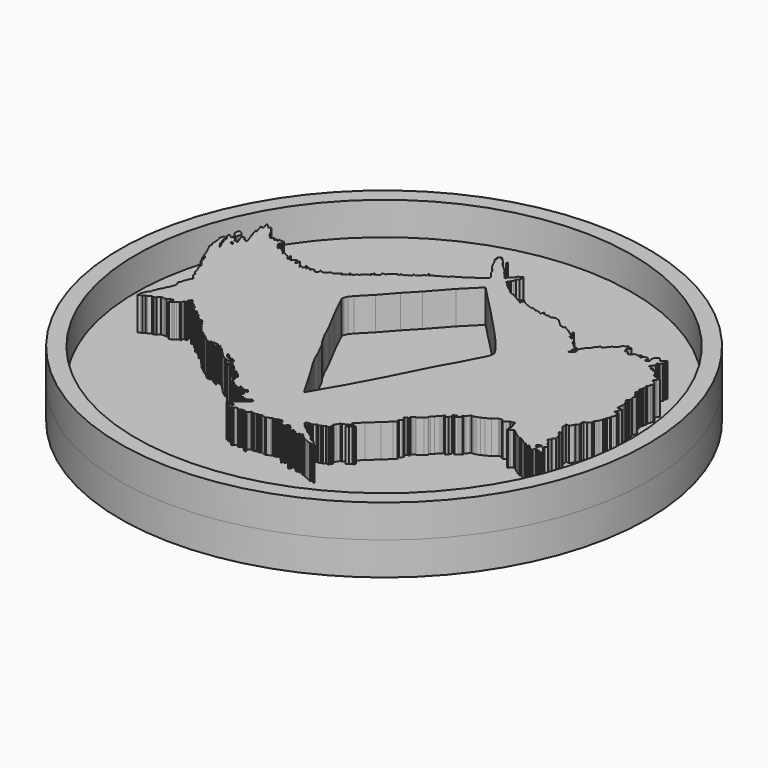
from build123d import *

# Parameters (mm, degrees)
F1_DEPTH = 2.5
F2_R     = 20
F2_R_2   = 18.8
F3_DEPTH = 2.5
F4_DEPTH = 2.5


with BuildPart() as f1:
    # F0 (on Top) → F1 (new body)
    with BuildSketch(Plane.XY):
        Polygon((2.8794382233, -10.7436152175), (2.8547642287, -10.5685461313), (2.8042409103, -10.7001410797), (2.7466679458, -10.7788639143), (2.7513678651, -10.8258621767), (2.7830917388, -10.8658103272), (2.835964784, -10.8705107123), (2.8770884965, -10.8364364132), (2.9052873142, -10.7906134799), align=None)
    extrude(amount=F1_DEPTH)


with BuildPart() as f1b:
    # F0 (on Top) → F1, piece 2 (new body)
    with BuildSketch(Plane.XY):
        Polygon((4.7097317874, -9.2714289203), (4.6033868566, -9.4176540151), (4.7296718694, -9.3312487006), (4.8094303347, -9.311308153), (4.9357153475, -9.1783767566), (5.0420602784, -9.1717308387), (5.1085259765, -9.0255057439), (4.9822414294, -9.0853255242), (4.9024824984, -9.1451443732), (4.7296718694, -9.1451443732), align=None)
    extrude(amount=F1_DEPTH)


with BuildPart() as f1c:
    # F0 (on Top) → F1, piece 3 (new body)
    with BuildSketch(Plane.XY):
        Polygon((2.7880056296, 9.804864414), (2.7621455956, 9.796067141), (2.7610280085, 9.7378306091), (2.7869136538, 9.7201569006), (2.831000369, 9.7271725535), (2.8474458959, 9.7436271608), (2.8180237859, 9.7701279446), (2.8097650502, 9.7977844998), align=None)
    extrude(amount=F1_DEPTH)


with BuildPart() as f1d:
    # F0 (on Top) → F1, piece 4 (new body)
    with BuildSketch(Plane.XY):
        Polygon((0.836121093, 10.7127986848), (0.8675596328, 10.6785539538), (0.9017927223, 10.6652751565), (0.9325326537, 10.6764575467), (0.9388203616, 10.7114007697), (0.9003954474, 10.7596227899), (0.842408801, 10.7596227899), align=None)
    extrude(amount=F1_DEPTH)


with BuildPart() as f1e:
    # F0 (on Top) → F1, piece 5 (new body)
    with BuildSketch(Plane.XY):
        Polygon((-1.0246526217, 12.8345778212), (-0.9706045967, 12.7852298319), (-0.9142065537, 12.7993291244), (-0.9165564552, 12.8392782062), (-0.9447555058, 12.8815760836), (-0.9447555058, 12.9191754386), (-0.9612049325, 12.9520744085), (-1.0035034502, 12.9497237504), (-1.0246526217, 12.9191754386), align=None)
    extrude(amount=F1_DEPTH)


with BuildPart() as f1f:
    # F0 (on Top) → F1, piece 6 (new body)
    with BuildSketch(Plane.XY):
        Polygon((-14.5434308797, 0.128211148), (-14.492415823, 0), (-14.3880443648, -0.1093972533), (-14.3209751695, -0.1149863165), (-14.3042076379, -0.1513153402), (-14.2622897401, -0.2239733585), (-14.2790572718, -0.3161931236), (-14.3628930673, -0.3720839159), (-14.3740717322, -0.475481851), (-14.4355511293, -0.6152088172), (-14.5193869248, -0.7884702063), (-14.5333595574, -0.9673206951), (-14.5764509216, -1.0409364477), (-14.6416602656, -1.1239300948), (-14.657468535, -1.1970434571), (-14.6495644003, -1.2780609541), (-14.5744746551, -1.3669827022), (-14.5329786465, -1.4598564012), (-14.5468106493, -1.5072813258), (-14.5626189187, -1.6139873769), (-14.615971595, -1.7187173944), (-14.6653726697, -1.8866806058), (-14.7167500108, -2.015122911), (-14.7878872231, -2.0585958846), (-14.8234562948, -2.2463193163), (-14.9084255099, -2.428114647), (-15.038844198, -2.5921256747), (-15.0783648714, -2.7245201636), (-15.0924259797, -2.8712532949), (-15.1289822534, -2.8579602949), (-15.1622146368, -2.8313740622), (-15.2020948008, -2.8513136785), (-15.1588916779, -3.017477924), (-15.1921240613, -3.1437624712), (-15.3383491561, -3.2833404839), (-15.3782283887, -3.3365131821), (-15.4181076214, -3.4860610031), (-15.5277764425, -3.635608824), (-15.4912201688, -3.7220141385), (-15.5011899769, -3.8383293431), (-15.5477160588, -3.9014716167), (-15.5443921685, -3.9479974657), (-15.4912201688, -3.9745839313), (-15.3649346903, -3.8782085758), (-15.2353271842, -3.8383293431), (-15.1223354042, -3.7087211385), (-15.0525458157, -3.6954279058), (-14.9960499257, -3.6854580976), (-14.7401569411, -3.5458800849), (-14.6770151332, -3.5624965094), (-14.6072255448, -3.5757897422), (-14.5174972713, -3.5359102767), (-14.4610013813, -3.4960308112), (-14.4277680665, -3.429565113), (-14.3181001768, -3.3331897575), (-14.2649272457, -3.2866639085), (-14.1153791919, -3.2833404839), (-14.0156811103, -3.2999569084), (-13.8694560155, -3.2866639085), (-13.6999692768, -3.1271460466), (-13.6401494965, -3.1304694712), (-13.6069171131, -3.1736721285), (-13.5570680723, -3.1637023203), (-13.5038951412, -3.1105296221), (-13.4440762922, -3.1204996631), (-13.4174898267, -3.1603788957), (-13.4141659364, -3.2235214021), (-13.4341064841, -3.2401378267), (-13.4407524019, -3.3298665658), (-13.5603910312, -3.4495047294), (-13.5304816067, -3.4760911949), (-13.3842565119, -3.3797158394), (-13.3344074711, -3.3464829903), (-13.2180927321, -3.3066035248), (-13.1350103766, -3.2334912103), (-13.0552519113, -3.1470858958), (-12.995432131, -3.087266814), (-12.9522299394, -3.0939131975), (-12.9322903231, -3.1271460466), (-12.9057038575, -3.1736721285), (-12.8525309265, -3.1603788957), (-12.8724705428, -3.0939131975), (-12.9057038575, -3.0407407321), (-12.8957340494, -2.9709516093), (-12.8458840773, -2.8679298703), (-12.7727724612, -2.8513134457), (-12.7428630367, -2.8978395276), (-12.7495089546, -2.9343955684), (-12.6558227235, -2.9278331026), (-12.593314983, -2.8679298703), (-12.6066077501, -2.7482914738), (-12.6597806811, -2.7549380902), (-12.7096297219, -2.7715545148), (-12.7395391464, -2.7449682821), (-12.7362161875, -2.6785025839), (-12.6996599138, -2.6186835021), (-12.6631036401, -2.5455711875), (-12.6099316403, -2.4957219139), (-12.5833451748, -2.449195832), (-12.5334952027, -2.4558424484), (-12.4969398603, -2.4890752975), (-12.4836461619, -2.5356013793), (-12.5235253945, -2.5389245711), (-12.5368190929, -2.5655108038), (-12.593314983, -2.5887738448), (-12.6199014485, -2.6220066939), (-12.593314983, -2.6352999266), (-12.5268492848, -2.631976502), (-12.5102326274, -2.6087134611), (-12.4305552999, -2.6058834381), (-12.3673314229, -2.6718562003), (-12.2144604102, -2.8313738294), (-12.1413478628, -2.8446670622), (-12.1081154794, -2.8778999113), (-12.1114384383, -2.9144559521), (-12.1546406299, -2.9709518421), (-12.1878739446, -3.017477924), (-12.1347010136, -3.064003773), (-12.1347010136, -3.1337928958), (-12.1147613972, -3.1537325121), (-12.0715592057, -3.1271462794), (-12.0449727401, -3.0507107731), (-11.9884768501, -2.9842450749), (-11.935303919, -2.9775984585), (-11.8721621111, -3.0540339649), (-11.8688382208, -3.1603791285), (-11.81898918, -3.246784443), (-11.7359068245, -3.3298665658), (-11.6528244689, -3.3996556886), (-11.5830358118, -3.4162721131), (-11.5464795381, -3.4362117294), (-11.5198930725, -3.4694445785), (-11.4866606891, -3.462798195), (-11.4999534562, -3.3930090722), (-11.4667210728, -3.3863624558), (-11.3636991009, -3.5060008522), (-11.2573541701, -3.5757897422), (-11.2772937864, -3.6555486731), (-11.3238198683, -3.7253377959), (-11.2939104438, -3.7851568777), (-11.2507073209, -3.7751868367), (-11.1975343898, -3.7186911795), (-11.1643020064, -3.7419542205), (-11.1410384998, -3.7652170286), (-11.0878665, -3.7652170286), (-11.0945133492, -3.7153677549), (-11.0612800345, -3.6954281386), (-11.0247237608, -3.7286609877), (-11.0180769116, -3.7652170286), (-11.0546331853, -3.7785102613), (-11.0579570755, -3.828359535), (-10.9914913774, -3.8748856168), (-11.0014611855, -3.9247348905), (-10.9017621726, -3.9513208903), (-10.8552360907, -3.9745839313), (-10.7854474336, -4.0476964787), (-10.762183927, -4.1208085604), (-10.6757786125, -4.2238305323), (-10.5926971883, -4.3202056549), (-10.5594638735, -4.3002660386), (-10.6026669964, -4.203890916), (-10.6093129143, -4.1374252178), (-10.5694336817, -4.0942225605), (-10.5262314901, -4.1008689441), (-10.473058559, -4.1540414095), (-10.3933000937, -4.180627875), (-10.3633897379, -4.2304769158), (-10.3301573545, -4.3334988877), (-10.260367766, -4.4398442842), (-10.1340832189, -4.5661288314), (-10.1565420628, -4.5993616804), (-10.1565420628, -4.6658483334), (-10.1012121886, -4.699440673), (-10.01821924, -4.7290814109), (-9.9846264347, -4.8002186231), (-9.8127108067, -5.0412951969), (-9.6091795713, -5.2369232289), (-9.5222331583, -5.2566835657), (-9.2080431059, -5.5333287455), (-9.1151697561, -5.5590169504), (-8.9116375893, -5.7329083793), (-8.6389444768, -5.9720091522), (-8.5974484682, -5.9720091522), (-8.5816401988, -5.9384163469), (-8.5381669924, -5.9403921477), (-8.484814316, -5.9897932224), (-8.4294844419, -5.9917694889), (-8.3823278546, -5.8678621426), (-8.3212293684, -5.872562062), (-8.3212293684, -5.9618586674), (-8.2648312673, -5.9665585868), (-8.1943338737, -5.8631622232), (-8.1285368651, -5.8584623039), (-8.0721378326, -5.914860405), (-8.0674383789, -5.9665585868), (-8.1097371876, -5.990057718), (-8.0909375101, -6.0605555773), (-8.001640439, -6.1451522633), (-7.8324470669, -6.2297494151), (-7.7337501571, -6.2908474356), (-7.7055511065, -6.2532485463), (-7.80894747, -6.0934540816), (-7.9828416929, -5.9383595362), (-7.9828416929, -5.9007611126), (-7.8653451055, -5.9007611126), (-7.8183468431, -5.9618586674), (-7.7337501571, -5.9994575568), (-7.6726521365, -6.0746548697), (-7.6323859394, -6.0681444593), (-7.6519171707, -5.9752599336), (-7.6116649434, -5.9836371802), (-7.5837196782, -6.0115824454), (-7.5390068814, -6.1177751049), (-7.3936907575, -6.1568985693), (-6.9968663156, -6.564901676), (-6.7118234001, -6.855533924), (-6.4491364174, -7.0455623791), (-6.3429442234, -7.1405768394), (-6.3094096258, -7.0790969767), (-6.0858465731, -7.1797003038), (-5.7999179699, -7.1964673698), (-5.5309436284, -7.3802778497), (-5.5260532536, -7.4194013141), (-5.5309436284, -7.4410592206), (-5.6119854562, -7.4389632791), (-5.653903354, -7.4655115604), (-5.709095858, -7.4704019353), (-5.7356436737, -7.4508399703), (-5.7649863884, -7.4061276391), (-5.7999179699, -7.4054286815), (-5.8292606845, -7.4277850799), (-5.8306581341, -7.5451559387), (-5.8250688016, -7.6003479771), (-5.7831509039, -7.6338825747), (-5.7272603735, -7.6303891838), (-5.6755612604, -7.605238352), (-5.6455200538, -7.5940601528), (-5.6301504374, -7.6101287268), (-5.571465008, -7.6799923554), (-5.5057932623, -7.7309925109), (-5.4603819735, -7.7344859019), (-5.4338336922, -7.7156224288), (-5.4345326498, -7.6632248238), (-5.4834363982, -7.621306926), (-5.54771116, -7.5500458479), (-5.5183684453, -7.5214020908), (-5.4750530981, -7.5144157745), (-5.3758467548, -7.512319833), (-5.3444080986, -7.5430595316), (-5.3139394149, -7.5977724046), (-5.249904003, -7.6606324874), (-5.1688319072, -7.7240802348), (-5.1406333223, -7.7693159692), (-5.0836475566, -7.8803496435), (-5.0025759265, -7.9884454608), (-4.9614524469, -8.0043077469), (-4.9326657318, -8.0184070393), (-4.9203289673, -8.0372067168), (-4.9044666812, -8.0389687791), (-4.8909545876, -8.0213444307), (-4.8850798048, -7.972584106), (-4.8551186919, -7.9396851361), (-4.8175198026, -7.9379221424), (-4.792845808, -7.9561341554), (-4.778158851, -8.0107701942), (-4.7975103371, -8.0780889839), (-4.8377527855, -8.1048198044), (-4.8565519974, -8.1059942022), (-4.8853382468, -8.0963009968), (-4.907369148, -8.0713331699), (-4.936743062, -8.0836704001), (-4.9438299611, -8.1195728853), (-4.9047064967, -8.139135316), (-4.8390347511, -8.1796552986), (-4.770568572, -8.2243680954), (-4.7230613418, -8.2634920254), (-4.6378280967, -8.3221774548), (-4.5623756014, -8.3976294845), (-4.5022927225, -8.4674935788), (-4.486923106, -8.5150003433), (-4.4533885084, -8.5122054443), (-4.4491966255, -8.4730824456), (-4.4575803913, -8.4185888991), (-4.503690172, -8.35012272), (-4.5595807023, -8.2844505087), (-4.6434169635, -8.202011697), (-4.7202669084, -8.1377374008), (-4.7188694589, -8.0762580037), (-4.6559926122, -8.0748600885), (-4.6294443309, -8.0874357373), (-4.5861289836, -8.139135316), (-4.503690172, -8.2257660106), (-4.4422103092, -8.277464658), (-4.3667578138, -8.3529166877), (-4.3360176496, -8.422780782), (-4.3304287829, -8.5122054443), (-4.3541821651, -8.5303699598), (-4.3835248798, -8.5331648588), (-4.4277254492, -8.552370593), (-4.4158692472, -8.5997954011), (-4.3714088388, -8.6156036705), (-4.3299118988, -8.6521608755), (-4.3200314976, -8.7035372853), (-4.3177357875, -8.746878244), (-4.3529844843, -8.751578629), (-4.3882331811, -8.7163290009), (-4.6349745244, -8.511886932), (-4.7877193429, -8.4413895383), (-4.9827625044, -8.2815950736), (-5.0274110399, -8.2839448005), (-5.0274110399, -8.3191934973), (-4.8464671709, -8.4766382352), (-4.6725734137, -8.5823843256), (-4.3703098781, -8.8347969577), (-4.3021366, -8.8476408273), (-4.2695323937, -8.8812336326), (-4.2626159266, -8.925694041), (-4.2952205986, -8.9622503147), (-4.2892927304, -9.0264715254), (-4.2398916557, -9.0610524639), (-4.1578859091, -9.0808132663), (-4.0986048989, -9.1163814068), (-3.9019891992, -9.2942258343), (-3.8259117864, -9.3149738386), (-3.7972591817, -9.3623986468), (-3.7942952476, -9.5007214695), (-3.7607026752, -9.5343142748), (-3.7172297016, -9.5293736085), (-3.6866010632, -9.4938054681), (-3.6895652302, -9.4483559951), (-3.7201938685, -9.4177275896), (-3.6698048934, -9.3940151855), (-3.6115117837, -9.4157522544), (-3.5275302362, -9.470093064), (-3.4484886564, -9.511590004), (-3.3674712759, -9.5679070801), (-3.2983098645, -9.5738349482), (-3.3081900328, -9.5382668078), (-3.3546269406, -9.4750327989), (-3.4020519815, -9.4078481197), (-3.4554048907, -9.3367109075), (-3.447500756, -9.2784175649), (-3.4010638483, -9.2803938314), (-3.3733993769, -9.3080578372), (-3.3338784706, -9.3495547771), (-3.3220222685, -9.3910517171), (-3.3368426375, -9.4384765252), (-3.3210343681, -9.470093064), (-3.2825015951, -9.470093064), (-3.2676812261, -9.4335367903), (-3.2874417957, -9.3801831827), (-3.2745974604, -9.3218907714), (-3.2370528206, -9.3544945121), (-3.214328317, -9.4167403877), (-3.1688795425, -9.4592245296), (-3.1619633082, -9.4888648018), (-3.1787597109, -9.5135653391), (-3.1836999115, -9.5600029454), (-3.1491192058, -9.5955710858), (-3.1184905674, -9.5679070801), (-3.1145385001, -9.5155416057), (-3.078969894, -9.478985332), (-3.0295688193, -9.4681167975), (-3.0107966159, -9.4434162602), (-2.9604076408, -9.4513203949), (-2.9554674402, -9.4809606671), (-2.922863001, -9.4918292016), (-2.8922343627, -9.4671286643), (-2.884330228, -9.4197038561), (-2.8457974549, -9.3762306497), (-2.7904682793, -9.3821594492), (-2.7446213644, -9.4327088445), (-2.7105624322, -9.4983885065), (-2.662953455, -9.553863667), (-2.6595285162, -9.6027906984), (-2.6643229648, -9.6385413781), (-2.7136956342, -9.6389073879), (-2.7333348989, -9.6118757501), (-2.7759657241, -9.5736039802), (-2.812409075, -9.5619810745), (-2.8387901839, -9.5730004832), (-2.8639938682, -9.5964064822), (-2.8681331314, -9.6304118633), (-2.8318210971, -9.6573270857), (-2.7942510787, -9.6872197464), (-2.7833986096, -9.7675379366), (-2.7471387293, -9.800334461), (-2.691736212, -9.8442640156), (-2.6922437828, -9.9030807614), (-2.7167205699, -9.9165057763), (-2.7269828133, -9.9915200844), (-2.7566659264, -10.013859719), (-2.7942019515, -10.0545044988), (-2.7952319942, -10.0997332484), (-2.7659838088, -10.1283127442), (-2.7263986412, -10.1476246491), (-2.6645348407, -10.185437277), (-2.6564844884, -10.2190319449), (-2.6371406857, -10.2809742093), (-2.5919666514, -10.3209223598), (-2.5399958249, -10.3163029999), (-2.4642604403, -10.2701280266), (-2.42394628, -10.2839870378), (-2.4239073973, -10.3422887623), (-2.4388970342, -10.3924917057), (-2.4225749075, -10.4381563142), (-2.3956054356, -10.436527431), (-2.3880430963, -10.3723956272), (-2.3656536359, -10.3390868753), (-2.330571413, -10.3345969692), (-2.3125640582, -10.3718852624), (-2.2290314082, -10.3759253398), (-2.2109330166, -10.3400908411), (-2.1629389375, -10.3387329727), (-2.1405748557, -10.3711355478), (-2.0698797889, -10.363153182), (-1.9555764738, -10.2994069457), (-1.896721893, -10.2260541171), (-1.8758515362, -10.1818563417), (-1.8310520099, -10.1755158976), (-1.7952256603, -10.2100688964), (-1.780948136, -10.2423671633), (-1.7529044999, -10.2412458509), (-1.7392452573, -10.2201765403), (-1.7106310697, -10.2156046778), (-1.6968038399, -10.2304108441), (-1.6927962424, -10.2660348639), (-1.6669204924, -10.2663682774), (-1.6629811144, -10.3098973632), (-1.6974124592, -10.3015489876), (-1.7234585248, -10.3209763765), (-1.6977177002, -10.3371180594), (-1.702507725, -10.3923929855), (-1.7546651652, -10.4391528293), (-1.87175069, -10.5127431452), (-1.932838466, -10.5949612334), (-2.0933183841, -10.6996148825), (-2.2541387007, -10.843789205), (-2.4408134632, -10.9487883747), (-2.5386204943, -11.0405934975), (-2.6165654417, -11.1426245421), (-2.6530593168, -11.168744415), (-2.6650137734, -11.1885322258), (-2.6334433351, -11.2072201446), (-2.5782184675, -11.2170716748), (-2.5484983344, -11.2407198176), (-2.5269410107, -11.2642636523), (-2.5344947353, -11.2990653142), (-2.5692218915, -11.3310245797), (-2.616596641, -11.3570038229), (-2.6545650326, -11.3440509886), (-2.7051893994, -11.3267805427), (-2.7573485859, -11.2762534991), (-2.8253407218, -11.2753771245), (-2.8591775335, -11.3090099767), (-2.8569214046, -11.3630490378), (-2.815447282, -11.3901728764), (-2.7519909199, -11.3918213174), (-2.6829980779, -11.3819083199), (-2.6343241334, -11.41577214), (-2.6230842341, -11.4790676162), (-2.5888672099, -11.5069290623), (-2.5434782729, -11.5008661523), (-2.4657761678, -11.4270830527), (-2.4158682209, -11.3421399146), (-2.3665726185, -11.3361282274), (-2.3199392017, -11.3209402189), (-2.2916600574, -11.3196428865), (-2.2644661367, -11.3391047344), (-2.2610439919, -11.365737766), (-2.274771221, -11.3713778555), (-2.3088706657, -11.4141469821), (-2.3202942684, -11.4713348448), (-2.309355652, -11.5794958547), (-2.2741658613, -11.6239888594), (-2.2062866483, -11.6846896708), (-2.1950600203, -11.7587875575), (-2.1678581834, -11.7774177343), (-2.1230611019, -11.7638697848), (-2.0963505376, -11.7326378822), (-2.0829422865, -11.656364426), (-2.0379344933, -11.6178914905), (-1.9482675707, -11.5824844688), (-1.7986700404, -11.5769337863), (-1.7790239071, -11.626210995), (-1.7375795869, -11.685741134), (-1.7186414916, -11.7109129205), (-1.6866568476, -11.7030153051), (-1.6800557496, -11.6773415357), (-1.6165057896, -11.6025451571), (-1.5781818656, -11.5997148678), (-1.5469130594, -11.5685435012), (-1.4283066848, -11.5617616102), (-1.4226280618, -11.5369064733), (-1.3916689204, -11.5422913805), (-1.3910334092, -11.5747051314), (-1.3666915474, -11.6082550958), (-1.3376430143, -11.623586528), (-1.3317067642, -11.5688210353), (-1.3259297702, -11.5323355421), (-1.2940651504, -11.5385623649), (-1.2915447587, -11.5643525496), (-1.2644589879, -11.5962773561), (-1.2034100946, -11.6020496935), (-1.1999645503, -11.6261914372), (-1.2420060812, -11.6372834891), (-1.2823358411, -11.6616915911), (-1.2764462736, -11.7199318483), (-1.2519740267, -11.7376977578), (-1.2157390593, -11.7664150894), (-1.1751411948, -11.8184564635), (-1.1380241485, -11.8505088612), (-1.0972052114, -11.8759628385), (-1.0562147945, -11.8814762682), (-1.0114887264, -11.876235716), (-0.9903045138, -11.8515808135), (-0.9909097571, -11.8150124326), (-1.0191196343, -11.8080014363), (-1.1096363887, -11.7278974503), (-1.0833578417, -11.6401575506), (-1.058412483, -11.6022555158), (-1.0243271245, -11.5611478686), (-0.9774729842, -11.5202050656), (-0.9389062179, -11.4882960916), (-0.9221833316, -11.4519502968), (-0.9200038039, -11.4096011966), (-0.8934841026, -11.400802061), (-0.8561364957, -11.4054372534), (-0.833510072, -11.4256711677), (-0.8410406299, -11.4538259804), (-0.8495628717, -11.4911077544), (-0.8169547655, -11.517287232), (-0.7504168316, -11.5206371993), (-0.6844786694, -11.4874178544), (-0.4738125717, -11.485144496), (-0.4214989603, -11.4451032132), (-0.3647063277, -11.4150904119), (-0.3384963202, -11.4428484812), (-0.3223508538, -11.4746317267), (-0.2886975708, -11.4850364625), (-0.257655367, -11.4804506302), (-0.2455709036, -11.4531852305), (-0.2161066514, -11.419496499), (-0.1647239551, -11.3819353282), (-0.0762701166, -11.3822445273), (-0.0345674307, -11.4110326394), (-0.0128800957, -11.4345774055), (0.0872699093, -11.453316547), (0.1590794564, -11.4808315411), (0.2412182512, -11.4727495238), (0.3274827613, -11.40821632), (0.4711195361, -11.353562586), (0.5765866372, -11.2826293334), (0.6623227964, -11.2804099917), (0.6876258412, -11.3073261455), (0.7323202444, -11.3062402233), (0.7553371834, -11.2799461931), (0.7784797344, -11.239528656), (0.81944064, -11.2483650446), (0.8393296157, -11.2685644999), (0.8794008754, -11.2748965621), (0.9114962304, -11.2537061796), (0.8834143518, -11.2317400053), (0.8610110381, -11.1849196255), (0.8765882812, -11.1759798601), (0.9139775066, -11.1756306142), (0.9777678642, -11.1806066707), (0.9931360837, -11.1965918913), (1.0340771405, -11.2079214305), (1.0724719614, -11.1967828125), (1.1148686754, -11.1433193088), (1.1677107541, -11.148984544), (1.2001374271, -11.1967660487), (1.3040129561, -11.2064126879), (1.3326881453, -11.2666077912), (1.3347847853, -11.3422498107), (1.2959734304, -11.3642485812), (1.2959734304, -11.4032393321), (1.3130656444, -11.4308791235), (1.3769947691, -11.4572355524), (1.4075816143, -11.4674111828), (1.4332249993, -11.5180499852), (1.4667029027, -11.5492260084), (1.4879414812, -11.5767493844), (1.4929594472, -11.6180386394), (1.5073154354, -11.6433771327), (1.5316131758, -11.6716390476), (1.546653104, -11.7067694664), (1.5720090596, -11.7008071393), (1.5770804603, -11.6449743509), (1.5568216331, -11.5923089907), (1.5441527357, -11.5488255396), (1.5612980351, -11.5162059665), (1.5874719247, -11.5039655939), (1.6103740782, -11.5161389112), (1.6045932425, -11.5649756044), (1.6342197778, -11.598196812), (1.6856824514, -11.5883797407), (1.7479301896, -11.5724112839), (1.7750544939, -11.5385232493), (1.7848344287, -11.4701744169), (1.8258518539, -11.4252846688), (1.8499820726, -11.3829728216), (1.8967994256, -11.3779865205), (1.9149947912, -11.402675882), (1.9532544538, -11.412252672), (1.9755812827, -11.4013608545), (1.9903734792, -11.3749988377), (2.0194663666, -11.3802654669), (2.0369400736, -11.4000542089), (2.0458565559, -11.4337084815), (2.0725447685, -11.4515200257), (2.0714821294, -11.4864427596), (2.0429727156, -11.5028452128), (2.0433743484, -11.546170339), (2.0568773616, -11.5812812001), (2.0873788744, -11.6019360721), (2.1430081688, -11.6431796923), (2.1669236012, -11.6260191426), (2.1153187845, -11.5624694154), (2.1193204448, -11.5422578529), (2.1599882748, -11.5392878652), (2.1766899154, -11.559067294), (2.2093774751, -11.5930270404), (2.2128811106, -11.7230350152), (2.2585373372, -11.7648486048), (2.2982556839, -11.7828277871), (2.3539855611, -11.8121933192), (2.3988650646, -11.8553936481), (2.3983621504, -11.9147794321), (2.3751542903, -11.9389351457), (2.3460180964, -11.9385598227), (2.3083202541, -11.9534470141), (2.3034969345, -11.9799356908), (2.3170770146, -12.0059633628), (2.3769652471, -11.9969528168), (2.4027100299, -11.9448797777), (2.4257835466, -11.9367921725), (2.4737427011, -11.8871014565), (2.469797153, -11.8094924837), (2.445789054, -11.7949787527), (2.4499809369, -11.7488689721), (2.482118085, -11.7069510743), (2.5659543462, -11.7090465501), (2.5959955528, -11.749567464), (2.6414068416, -11.7803076282), (2.7147633955, -11.7831015959), (2.7594761923, -11.8201291189), (2.776941983, -11.8536641821), (2.8020928148, -11.9053637609), (2.8502985369, -11.9563639164), (2.9089839663, -11.9975833222), (2.9809433036, -11.9968848303), (3.0039981939, -11.9731305167), (3.0158751179, -11.9207333773), (3.0508066993, -11.8858013302), (3.0759575311, -11.8396915495), (3.1213688198, -11.828513816), (3.1597937923, -11.8348011747), (3.16887605, -11.8592530489), (3.136738902, -11.8823079392), (3.100409871, -11.9214318693), (3.140930552, -11.9731305167), (3.1968213152, -11.9598563761), (3.2191777136, -11.8927871808), (3.2897398341, -11.8438834324), (3.2799588516, -11.8138417602), (3.2436300535, -11.7810061201), (3.3079043496, -11.7726223543), (3.3735760953, -11.8501707911), (3.3945350442, -11.9333080947), (3.5022012889, -11.9918836281), (3.4528530668, -12.0388818905), (3.4575529862, -12.0788309723), (3.5022012889, -12.1023301035), (3.5562494304, -12.0388818905), (3.600897966, -12.0435822755), (3.600897966, -12.0905805379), (3.683145158, -12.1634276584), (3.7324933801, -12.175177224), (4.0779314004, -12.330272235), (4.1719279252, -12.3467212543), (4.2330259457, -12.4031193554), (4.3364223093, -12.4524673447), (4.4327690266, -12.389020063), (4.7006593086, -12.5182652846), (4.7147590667, -12.4971158803), (4.5526148751, -12.3373214155), (4.4025308453, -12.1875908226), (4.286557436, -12.0702199638), (4.2460365221, -12.0296990499), (4.2125023901, -11.9975619018), (4.2013241909, -12.0324939489), (4.1901459917, -12.0841925964), (4.0769670159, -12.028302066), (4.0085008368, -11.9752055034), (3.927459009, -11.8690133095), (3.8883355446, -11.8159167469), (3.8841438945, -11.6985458881), (3.9218701422, -11.669203639), (3.9260620251, -11.6230938584), (3.8939246442, -11.6077233106), (3.8464176469, -11.6356695071), (3.8296503481, -11.6831762716), (3.7360333372, -11.6747925058), (3.6466079764, -11.6147100925), (3.5753473639, -11.5420520306), (3.3112633973, -11.3953389227), (3.1617556233, -11.2500227988), (3.0863031279, -11.1745707691), (2.9898914509, -11.1298579723), (2.8906853404, -11.0613917932), (2.8753154911, -11.0250627622), (2.9088498559, -10.9901307151), (2.89627444, -10.9076919034), (2.8417808935, -10.9160756692), (2.815232845, -10.9649803489), (2.7691230644, -10.9663773328), (2.7230130509, -10.9314452857), (2.6573413052, -10.8420206234), (2.6238069404, -10.7428142801), (2.5525460951, -10.7232527807), (2.4575316347, -10.6128687039), (2.4673126172, -10.53322386), (2.5427651126, -10.4661546648), (2.6349849068, -10.4382093996), (2.6852865703, -10.394894518), (2.7272047009, -10.3976884857), (2.7313965838, -10.4396063834), (2.7383829001, -10.5583751574), (2.7579446323, -10.5835255235), (2.787287347, -10.5583751574), (2.8040546458, -10.4857170954), (2.8669317253, -10.4200448841), (2.9004660901, -10.4200448841), (2.9144389555, -10.4493880644), (2.9675350524, -10.4451961815), (3.1212347094, -10.2803185582), (3.1980846543, -10.2621540427), (3.2176463865, -10.3096608073), (3.2875097822, -10.3040719405), (3.3881133422, -10.2230301127), (3.4551820718, -10.2188382298), (3.4761412535, -10.2453865111), (3.5725529306, -10.2286189795), (3.6759506911, -10.1028652862), (3.7625813857, -10.0860977545), (3.833842231, -10.1419882849), (3.8827466778, -10.1280156523), (3.8869385608, -10.0805088878), (3.9330483414, -10.0218234584), (3.9274594747, -9.9491653964), (4.00291197, -9.9449735135), (4.0238709189, -9.890479967), (3.9484184235, -9.8164249212), (3.8967193104, -9.718616493), (3.8995139766, -9.6515472978), (4.0126927197, -9.5537388697), (4.1440362111, -9.3231890351), (4.250228405, -9.3176001683), (4.4081201777, -9.2058181763), (4.4360654429, -9.2700924724), (4.5254910365, -9.182064794), (4.6386695467, -9.1024199501), (4.7434647568, -9.0968310833), (4.7797937877, -9.0493233874), (4.7197113745, -9.0185841545), (4.6749985777, -8.9235696942), (4.7079001818, -8.7904037561), (5.206303671, -8.3300461993), (5.9009861243, -7.6702110477), (6.4279139042, -7.1835066192), (6.610956043, -7.014437113), (6.6025727428, -6.9424775429), (6.5529695712, -6.9026555866), (6.5543670207, -6.7943669856), (6.7080669105, -6.6672158428), (6.7499848083, -6.6106263548), (6.755573675, -6.5142144449), (6.5941894427, -6.4240903594), (6.6004772671, -6.3716927543), (6.7674508318, -6.2508285046), (6.8687526509, -6.2389518134), (6.9253421389, -6.1795678921), (6.9393147714, -6.1586089432), (6.9148628972, -6.1404444277), (6.847793702, -6.1229784042), (6.8554785103, -6.0817589983), (6.9064791314, -6.0461289249), (6.9546848536, -5.9727719054), (7.0534395054, -5.9045953676), (7.1260975674, -5.8682663366), (7.1579422802, -5.9026554227), (7.5341002084, -5.6167580187), (7.693388965, -5.4714418948), (7.7269230969, -5.3904005326), (7.6654432341, -5.3680441342), (7.6654432341, -5.33730397), (7.7353068627, -5.2730296738), (7.916951552, -5.1333028823), (8.1385448575, -4.8903045245), (8.2278419286, -4.801007919), (8.2912901416, -4.7023114748), (8.3594378084, -4.6647125855), (8.4205353633, -4.6811620705), (8.4369843826, -4.725810606), (8.4134852514, -4.7916080803), (8.4698833525, -4.8057078384), (8.5192322731, -4.7775087878), (8.6273280904, -4.6882117167), (8.6555276066, -4.6059647575), (8.6954757571, -4.5519163832), (8.7166251615, -4.4626197778), (8.6884256452, -4.3968218379), (8.6672771722, -4.3310243636), (8.8035715744, -4.2511271313), (8.911668323, -4.213528242), (8.9563168585, -4.2323279195), (8.9234178886, -4.2981253937), (8.8693695143, -4.4062216766), (8.8623203337, -4.4649695046), (8.9234178886, -4.4626197778), (9.0855611488, -4.3427739292), (9.1678090394, -4.2581767775), (9.2947045341, -4.1735796258), (9.3088038266, -4.1359812021), (9.2571051791, -4.138330929), (9.2077571899, -4.1477307677), (9.1748582199, -4.138330929), (9.1490093619, -4.1030822322), (9.1560594738, -4.0537337773), (9.2030577362, -3.9996858686), (9.3581518158, -3.9174389094), (9.4826975837, -3.7576442119), (9.5743443817, -3.689496778), (9.7435377538, -3.6847968586), (9.8915826529, -3.6377985962), (10.135974735, -3.5532014444), (10.3850653395, -3.4357055556), (10.7399029657, -3.2477120403), (11.0571421683, -2.9821712524), (11.12058945, -2.9586721212), (11.2451352179, -2.9657220002), (11.3132828847, -2.9539722018), (11.367331259, -2.9892211314), (11.3861300051, -3.0409193132), (11.4049296826, -3.0714680906), (11.4613277838, -3.0879175756), (11.5200756118, -3.0738180503), (11.6258217022, -2.9915710911), (11.7715168744, -2.8693752829), (11.8373148143, -2.8341265861), (11.9900591671, -2.836476313), (12.1028553694, -2.8247267473), (12.1545530856, -2.7871280909), (12.1898027137, -2.7988776565), (12.1921524405, -2.8388262726), (12.1639529243, -2.9210734647), (12.1663026512, -2.9986207373), (12.2415004298, -3.0244698282), (12.2908484191, -3.1701647677), (12.3448967934, -3.3229093533), (12.3495962471, -3.4780038986), (12.3002482578, -3.499153303), (12.264999561, -3.5673007369), (12.3448967934, -3.656597808), (12.3448967934, -3.7834933028), (12.3848449439, -3.8328415249), (12.4388933182, -3.8187419996), (12.4647421762, -3.7435446866), (12.5234900042, -3.6683473736), (12.6456860453, -3.5837502219), (12.7091342583, -3.557901131), (12.7678820863, -3.574350616), (12.8853777424, -3.6824468989), (13.0992205814, -3.8492910098), (13.2754640654, -3.9691366255), (13.5151557624, -4.1148317978), (13.5927032679, -4.1430308484), (13.6232515797, -4.1312812828), (13.6937499046, -4.1265813634), (13.9006730169, -4.2631248944), (14.0753323212, -4.401454702), (14.2010860145, -4.4587426819), (14.2639633268, -4.4769071974), (14.3264252692, -4.4465810061), (14.346987009, -4.4689052738), (14.3483411521, -4.4816131704), (14.4155258313, -4.5606545173), (14.4649269059, -4.5863431878), (14.5163042471, -4.6159834601), (14.5854651928, -4.6258638613), (14.6407941356, -4.5487983152), (14.6803148091, -4.5784390531), (14.7672602907, -4.6396963298), (14.8522304371, -4.7503542155), (14.9826491252, -4.8155635595), (15.0715708733, -4.8985569738), (15.1268998161, -4.8689167015), (15.1348039508, -4.7701145522), (15.1427080855, -4.6495762654), (15.1664204895, -4.5883189887), (15.2355814353, -4.5883189887), (15.2869587764, -4.6159834601), (15.3225269169, -4.6535283327), (15.3561197221, -4.6772407368), (15.4193527997, -4.6811928041), (15.5161786824, -4.7266418114), (15.5774364248, -4.764186684), (15.6189324334, -4.8096352257), (15.6545024365, -4.8116114922), (15.6703107059, -4.7878990881), (15.6861189753, -4.764186684), (15.6999509782, -4.8116114922), (15.7710872591, -4.7681387514), (15.7453995198, -4.6495762654), (15.7118067145, -4.5744869858), (15.545819886, -4.3749068864), (15.4648022726, -4.3057459407), (15.4252815992, -4.256344866), (15.4151087627, -4.1462080553), (15.4715068638, -4.1368086822), (15.6360007823, -4.0099127218), (15.5937029049, -3.915916197), (15.377510339, -3.7561217323), (15.3305120766, -3.6527253687), (15.2459153906, -3.5117303487), (15.1801174507, -3.4130339045), (15.0908203796, -3.3848348539), (15.0250224397, -3.3331366722), (15.0156235322, -3.2720386516), (15.0720207021, -3.2062411774), (15.1715520769, -3.1211215537), (15.1250259951, -3.0745954718), (15.0917936116, -3.02806939), (15.1715520769, -2.981543541), (15.3310699388, -2.8619051445), (15.1914916933, -2.4431713391), (15.0851467624, -2.2903000936), (14.9854486808, -2.2238343954), (14.9189829826, -2.1573686972), (14.9721549824, -2.0842563827), (15.051914379, -2.0709631499), (15.1250259951, -2.0443769172), (15.0386206806, -1.8981524045), (14.6597661078, -1.4195992844), (14.666412957, -1.3066076208), (14.6797057241, -1.2202021899), (14.6398264915, -1.1537363753), (14.6597661078, -1.0872706771), (14.7195858881, -1.0739775607), (14.8791028187, -1.0806241771), (15.0585602969, -0.8413475589), (15.0917936116, -0.7150627207), (15.1724535972, -0.644225569), (15.2674680576, -0.5548003246), (15.2339339256, -0.4541969392), (15.2115775272, -0.3759497777), (15.289824456, -0.2865245333), (15.2339339256, -0.2474010398), (15.2618791908, -0.174743036), (15.4574969783, -0.1244412706), (15.5413327739, -0.0182488347), (15.6195806339, 0.0544091672), (15.6810600311, 0.0935327407), (15.7201830298, 0.2276706073), (15.6810600311, 0.2444378624), (15.6698822975, 0.272383244), (15.7034154981, 0.2891504846), (15.7648958266, 0.3618084884), (15.8599112183, 0.5462480476), (15.9772820771, 0.7586330175), (15.9325692803, 0.7865783991), (15.9213896841, 0.8312910213), (16.0164050758, 0.9263053653), (16.0164050758, 1.1051559122), (16.1337759346, 1.2169374386), (16.1058306694, 1.3622534461), (16.1952544004, 1.4908022713), (16.2679124624, 1.6025837976), (16.3126252592, 1.66965276), (16.2902697921, 1.7423107056), (16.2455569953, 1.7255435232), (16.1728989333, 1.7478998052), (16.1784887314, 1.8149687676), (16.2064339966, 1.8764486304), (16.1561314017, 1.9379284931), (16.1617211998, 2.0105864387), (16.0275828093, 1.9770520739), (15.8766768873, 1.9658738747), (15.8375538886, 2.0049973391), (15.9493349493, 2.1503134631), (15.9925278276, 2.3548081517), (16.0489268601, 2.4582045153), (15.9502308816, 2.4535048287), (15.8985313028, 2.5334020611), (15.8280339092, 2.4958034046), (15.7152377069, 2.4629044347), (15.6823396683, 2.5381017476), (15.6964398921, 2.7871930506), (15.7340373844, 2.9610870406), (15.7011393458, 3.10678198), (15.6588405371, 3.2289775554), (15.6400408596, 3.2994751818), (15.687039122, 3.332373919), (15.6917385757, 3.4216709901), (15.7528370619, 3.4216709901), (15.7951358706, 3.4686692525), (15.7622359693, 3.5485664848), (15.6964398921, 3.572065616), (15.6212411821, 3.5250673536), (15.5460443348, 3.4733691718), (15.4849467799, 3.4874686971), (15.4708465561, 3.5532664042), (15.536644496, 3.6284637172), (15.6212411821, 3.7318600807), (15.6353414059, 3.8352564443), (15.6053351238, 3.96407675), (15.5630363151, 4.0157749318), (15.5865354463, 4.0674731135), (15.5959352851, 4.1802693158), (15.6382340938, 4.2648664676), (15.661733225, 4.354163073), (15.6288351864, 4.3823621236), (15.5724361539, 4.3682628311), (15.5395371839, 4.3353638612), (15.5160380527, 4.3729622848), (15.506638214, 4.4481600635), (15.4549404979, 4.4481600635), (15.4032418504, 4.4951583259), (15.4173420742, 4.5844549313), (15.3844431043, 4.6549527906), (15.3045458719, 4.6361531131), (15.271646902, 4.6831518412), (15.2951460332, 4.7348500229), (15.3186451644, 4.7959475778), (15.3421442956, 4.8805447295), (15.3186451644, 4.9698418006), (15.3233446181, 5.0591384061), (15.2481477708, 5.0638383254), (15.2481477708, 5.1014372148), (15.271646902, 5.1296362653), (15.2763463557, 5.2001336589), (15.2904465795, 5.3082299419), (15.3280450031, 5.3552282043), (15.3515441343, 5.3928266279), (15.3186451644, 5.4210256785), (15.3182623908, 5.4731206037), (15.3322350234, 5.509449169), (15.3769478202, 5.601669196), (15.3713589534, 5.6827110238), (15.309878625, 5.6407926604), (15.273549594, 5.637998227), (15.2987008914, 5.7386015542), (15.3713589534, 5.8475886472), (15.4076879844, 5.9593701735), (15.4412221164, 6.0655628331), (15.4887298122, 6.1577823944), (15.4831400141, 6.2416186556), (15.424455516, 6.3226600178), (15.3266461566, 6.4316471107), (15.2707556263, 6.5015107393), (15.2148650959, 6.4987163059), (15.1785360649, 6.4735654742), (15.1394121349, 6.4903325401), (15.1505898684, 6.5853470005), (15.2600212023, 6.7459307611), (15.300530009, 6.8091638386), (15.3855001554, 6.8812891841), (15.3489429504, 6.9089536555), (15.3153501451, 6.9178459235), (15.2649618685, 6.8980855867), (15.18888399, 6.9010495208), (15.1098426431, 6.9534145296), (15.02586063, 6.9879954681), (14.9310110137, 6.9978754036), (14.8559221998, 7.0245517418), (14.8025685921, 7.0680249482), (14.7620597854, 7.1292817593), (14.7255035117, 7.2043715045), (14.6800549701, 7.3199695908), (14.6385580301, 7.3851789348), (14.5990373567, 7.4158073403), (14.5506244153, 7.4503878132), (14.5111037418, 7.4691604823), (14.5012233406, 7.4958368205), (14.5150553435, 7.5126332231), (14.5190078765, 7.5373337604), (14.5081393421, 7.5689502992), (14.4696068019, 7.5827827677), (14.4478706643, 7.5738904998), (14.414277859, 7.5511657633), (14.353021048, 7.5037409551), (14.3283205107, 7.5017651543), (14.3065834418, 7.5284414925), (14.2947277054, 7.5482018292), (14.3036199734, 7.5709261), (14.3065843731, 7.63317151), (14.2749678344, 7.6647880487), (14.2403868958, 7.6815844513), (14.2305064946, 7.6815844513), (14.1860460863, 7.6400879771), (14.1208367422, 7.6025431044), (14.087243937, 7.61242304), (14.1030522063, 7.645027712), (14.1228130087, 7.6756565832), (14.1366450116, 7.7112251893), (14.1010759398, 7.7270334587), (14.0576036647, 7.7388896607), (14.0190711245, 7.772482466), (13.9825139195, 7.8001469374), (13.9716463163, 7.8228712082), (13.9341009781, 7.8307753429), (13.9094004408, 7.8120031394), (13.8758076355, 7.7922428027), (13.8175152242, 7.7971825376), (13.8017069548, 7.8327516094), (13.8352988288, 7.8732604161), (13.8866761699, 7.9177208245), (13.9123639092, 7.9730497673), (13.9439804479, 8.0125704408), (13.9874536544, 8.0748163164), (14.0299377963, 8.120264858), (14.0605671331, 8.1558339298), (14.0566146001, 8.1933783367), (13.9795495197, 8.297120221), (13.9775732532, 8.394934237), (14.004250057, 8.4216110408), (14.032902196, 8.4453234449), (14.0556273982, 8.4453234449), (14.0852676705, 8.423586376), (14.1277527437, 8.4225991741), (14.148500748, 8.4502631798), (14.1761656851, 8.4848441184), (14.1969136894, 8.5520287976), (14.2482910305, 8.624154143), (14.2522426322, 8.6923278868), (14.2216142267, 8.7476568297), (14.2067931592, 8.7970579043), (14.209757559, 8.8316379115), (14.2374224961, 8.8602909818), (14.279906638, 8.9096920565), (14.2818829045, 8.9907087386), (14.2571823671, 9.0243015438), (14.2156854272, 9.0154092759), (14.1870332882, 8.9877452701), (14.0941590071, 8.9166080579), (13.9844892547, 8.8227456436), (13.9607768506, 8.7911291048), (13.9360763133, 8.7664285675), (13.910388574, 8.7674167007), (13.8916159049, 8.7901409715), (13.8817355037, 8.8138533756), (13.8520952314, 8.8257100433), (13.8105982915, 8.8513987139), (13.7750292197, 8.898823522), (13.7444008142, 8.9442720637), (13.705868274, 8.9847808704), (13.6831440032, 9.0075051412), (13.6564671993, 9.0243015438), (13.6218862608, 9.0183736756), (13.59916199, 9.0005900711), (13.5724851862, 8.9719370008), (13.5102402419, 8.9225359261), (13.4450308979, 8.8602909818), (13.3926654235, 8.8029857725), (13.3778452873, 8.7654413655), (13.3778462186, 8.6587360129), (13.3462296799, 8.5698142648), (13.4361395612, 8.4552029148), (13.4341632947, 8.3751734346), (13.373894617, 8.3178682253), (13.2988048717, 8.2378387451), (13.2187753916, 8.2279592752), (13.162988238, 8.2574216649), (13.1383147091, 8.2785710692), (13.1465392187, 8.309119381), (13.1676886231, 8.3373188972), (13.2123371586, 8.3831418306), (13.2240867242, 8.4383655339), (13.2170366123, 8.497113362), (13.166513294, 8.5593862459), (13.0948405713, 8.5969846696), (13.0125936121, 8.6063845083), (12.9409208894, 8.5899345577), (12.893922627, 8.5617359728), (12.8234252334, 8.526487276), (12.7834770828, 8.4841884673), (12.7646774054, 8.4160408005), (12.7223785967, 8.3854924887), (12.6706808805, 8.3725675941), (12.6213328913, 8.4078162909), (12.6107577235, 8.4442403167), (12.6460064203, 8.4665641189), (12.6730306074, 8.5147377104), (12.6753803343, 8.5734855384), (12.6460064203, 8.5981599987), (12.5790340826, 8.5946349427), (12.5390850008, 8.5511617362), (12.4744623899, 8.4700891748), (12.3910401016, 8.4712645039), (12.3510919511, 8.526487276), (12.291168794, 8.5253119469), (12.2829442844, 8.5065132007), (12.2053967789, 8.4912385792), (12.1384244412, 8.4477653727), (12.1254995465, 8.3666928113), (12.0773268864, 8.3396695554), (11.9856800884, 8.317344822), (11.9281066582, 8.2538975403), (11.8305850774, 8.2703465596), (11.7777120322, 8.317344822), (11.754212901, 8.4031168371), (11.7072146386, 8.4512904286), (11.5932431072, 8.4536401555), (11.515696533, 8.4219165146), (11.4804469049, 8.4536401555), (11.4827975631, 8.5159130394), (11.5180462599, 8.5676116869), (11.4992465824, 8.5887601599), (11.4075997844, 8.5911098868), (11.3864503801, 8.6181340739), (11.3876257092, 8.6674820632), (11.4252241328, 8.7180053815), (11.5004219115, 8.7885027751), (11.548595503, 8.8366763666), (11.5920687094, 8.8801495731), (11.6132181138, 8.9048240334), (11.5944184363, 8.9330226183), (11.5732690319, 8.9635718614), (11.5227457136, 8.9635718614), (11.5062966943, 8.9471219108), (11.4839728922, 8.9142238721), (11.4534236491, 8.8930744678), (11.4369736984, 8.8742747903), (11.4052500576, 8.8707497343), (11.3794011995, 8.8954241946), (11.3488519564, 8.9212730527), (11.3488519564, 8.970621042), (11.3371023908, 9.0246694162), (11.3030290231, 9.0493438765), (11.2677803263, 9.0575683862), (11.2243061885, 9.0223196894), (11.1937578768, 8.9717973024), (11.1655592918, 8.9200986549), (11.1115109175, 8.8637005538), (11.0868364573, 8.8637005538), (11.0891871154, 8.895425126), (11.0574625432, 8.9259734377), (11.0468883067, 8.8965995237), (11.0092898831, 8.8543016464), (10.9611162916, 8.8108275086), (10.9141180292, 8.7438551709), (10.890618898, 8.6439838633), (10.849494487, 8.5640866309), (10.7766473666, 8.5253128782), (10.6826508418, 8.4677403793), (10.6168529019, 8.4383664653), (10.5369556695, 8.4242662415), (10.5099314824, 8.3619933575), (10.4641085491, 8.2891462371), (10.3278141469, 8.1328768283), (10.2655412629, 8.0670788884), (10.2126682177, 8.0165555701), (10.1633192971, 7.9789571464), (10.1280706003, 7.9401833937), (10.0798979402, 7.9460581765), (10.0798979402, 7.994231768), (10.0375991315, 7.994231768), (9.9812010303, 7.9472335055), (9.9107036367, 7.8743854538), (9.8143564537, 7.7592399903), (9.7368098795, 7.646443788), (9.6698366106, 7.5207236223), (9.6275378019, 7.4396515265), (9.5711397007, 7.3726787232), (9.4982925802, 7.3104058392), (9.4242701307, 7.2622327134), (9.3549471349, 7.1741109714), (9.2679997906, 6.9943424314), (9.1986777261, 6.8756714463), (9.1881025583, 6.6841533408), (9.2069022357, 6.6395048052), (9.2186518013, 6.5983813256), (9.2480257154, 6.616005674), (9.2738745734, 6.645379588), (9.2832744122, 6.6124806181), (9.2738745734, 6.5513825975), (9.2527251691, 6.524358876), (9.2245265841, 6.4926347695), (9.1881025583, 6.4597357996), (9.1317044571, 6.41861232), (9.0870559216, 6.3821887597), (9.0518072248, 6.3398899511), (9.0036336333, 6.268217694), (8.9625101537, 6.2329689972), (8.9225620031, 6.2317941338), (8.9284367859, 6.2611680478), (8.9554609731, 6.3163908198), (8.9860092849, 6.3868886791), (9.0012839064, 6.4585609362), (8.9766094461, 6.5302336589), (8.9354859665, 6.6019059159), (8.9895352721, 6.7217517644), (8.9848348871, 6.8039987236), (8.9930593967, 6.9073950872), (9.021258913, 6.9485190324), (9.0059842914, 6.9908173755), (8.9660361409, 6.9896425121), (8.9401863515, 6.959093269), (8.9225620031, 6.9085704163), (8.8191656396, 6.9849425927), (8.7510179728, 7.0366407745), (8.657021448, 7.0883389562), (8.61160364, 7.1785622276), (8.5562746972, 7.231914904), (8.5108261555, 7.2516752407), (8.4535209462, 7.2793401778), (8.4159756079, 7.3425732553), (8.4219044074, 7.4097584002), (8.4475921467, 7.4571832083), (8.4140002728, 7.4848476797), (8.3764549345, 7.5263446197), (8.3389105275, 7.5283208862), (8.3191497251, 7.5006559491), (8.2816053182, 7.4986801483), (8.2835815847, 7.5955060311), (8.2618454471, 7.6587391086), (8.2183722407, 7.7061639167), (8.1926835701, 7.7437087893), (8.1571154296, 7.7634691261), (8.0978339538, 7.7733495273), (8.0760978162, 7.8089181334), (8.066217415, 7.8306542709), (8.0326246098, 7.8187985346), (8.0266967416, 7.7753253281), (8.0089122057, 7.7298763208), (7.9674152657, 7.7358046547), (7.9298708588, 7.7911335975), (7.8863976523, 7.8365821391), (7.8547811136, 7.8326305375), (7.833044976, 7.8010139987), (7.8073563054, 7.7970619313), (7.7856201679, 7.8247264028), (7.7717876993, 7.9215522856), (7.7540031634, 7.9808337614), (7.7777155675, 8.0124503002), (7.7599314973, 8.0756833777), (7.7421469614, 8.0974195153), (7.7026262879, 8.0816112459), (7.6690334827, 8.1171803176), (7.6868180186, 8.1567009911), (7.7243624255, 8.2159815356), (7.7362190932, 8.2831671461), (7.7125062235, 8.3365207538), (7.6492731459, 8.403705433), (7.6038241386, 8.403705433), (7.5998720713, 8.3246640861), (7.6255607419, 8.273286745), (7.6393932104, 8.2140062004), (7.6156808063, 8.1626288593), (7.5544235297, 8.1606525928), (7.493166253, 8.2001732662), (7.4358615093, 8.2673588768), (7.3706521653, 8.296999149), (7.2975386865, 8.3681372926), (7.2046648711, 8.3780167624), (7.0367017761, 8.5163395852), (6.9398758933, 8.5440045223), (6.8667624146, 8.6250221357), (6.8173618056, 8.6349016055), (6.7995772697, 8.6092138663), (6.7956252024, 8.5598127916), (6.7778406665, 8.5459798574), (6.7482003942, 8.5459798574), (6.7363441922, 8.5874767974), (6.6987993196, 8.5894530639), (6.6652065143, 8.5361003876), (6.6493982449, 8.5341241211), (6.6316141747, 8.571668528), (6.5841893665, 8.6230458692), (6.5387403592, 8.6210696027), (6.5347882919, 8.571668528), (6.505147554, 8.571668528), (6.4636510797, 8.6013097316), (6.3035916537, 8.8008893654), (6.2522147782, 8.8068172336), (6.1711971648, 8.887834847), (5.9696417302, 9.0972948819), (5.8629354462, 9.1071752831), (5.7483254932, 9.1763362288), (5.6440723129, 9.1931512579), (5.6045558304, 9.1595528647), (5.5131330155, 9.1678434983), (5.4361349903, 9.148507379), (5.3997337818, 9.097953327), (5.3515420295, 9.080353193), (5.2851201035, 9.0686520562), (5.2580470219, 9.0975034982), (5.2403644659, 9.1428169981), (5.2074198611, 9.1646155342), (5.130992271, 9.1629270464), (5.0957375206, 9.1423736885), (5.0422712229, 9.1077191755), (4.9881795421, 9.1113019735), (4.9105505459, 9.1360853985), (4.8335120082, 9.1579267755), (4.7929314896, 9.1714970767), (4.7717210837, 9.2174028978), (4.7334493138, 9.2750899494), (4.6957707964, 9.3274815008), (4.6569551341, 9.3404622748), (4.6334550716, 9.323425591), (4.6305353753, 9.3040158972), (4.6499501914, 9.2898793519), (4.6982136555, 9.2357108369), (4.6999990009, 9.2139448971), (4.6947193332, 9.2021841556), (4.6171182767, 9.1981422156), (4.5894985087, 9.1858161613), (4.5995255932, 9.1534517705), (4.6371864155, 9.1187069193), (4.641356878, 9.0634077787), (4.58667567, 9.0681677684), (4.532547202, 9.1088106856), (4.4725742191, 9.1135771945), (4.4325781055, 9.1318525374), (4.3786405586, 9.1928411275), (4.3255076744, 9.1900946572), (4.2807864957, 9.164955467), (4.2276009917, 9.2153763399), (4.1856402531, 9.2266108841), (4.1800695471, 9.2042302713), (4.1101677343, 9.1903088614), (3.8387342356, 9.3528758734), (3.7800027058, 9.3557322398), (3.7828739733, 9.2801777646), (3.7297382951, 9.28023085), (3.6122021265, 9.3586975709), (3.4891506657, 9.3588205054), (3.380021546, 9.4204898924), (3.2821204513, 9.4401743263), (2.9575258959, 9.6279783174), (2.8959671035, 9.6616186202), (2.8120656498, 9.6645001322), (2.8148873243, 9.6393125132), (2.8400681913, 9.6280956641), (2.8457057197, 9.5833176747), (2.8149429709, 9.5833484083), (2.6721456088, 9.7541827708), (2.6246253401, 9.7318440676), (2.6302880142, 9.6618821844), (2.7926363982, 9.5162121579), (2.7843324933, 9.4294762239), (2.7200051118, 9.4351358712), (2.5940069463, 9.5863658935), (2.4960890878, 9.6228402108), (2.420613775, 9.5893368125), (2.3058354855, 9.7069758922), (2.2079397459, 9.7210649401), (2.1328052174, 9.8027516563), (2.0339831244, 9.8248878494), (1.9774872344, 9.9279088899), (1.5620766208, 10.0209610537), (1.2995370198, 10.2635612711), (1.0469673434, 10.4463417083), (0.917359197, 10.5693032965), (0.7877510507, 10.655708611), (0.6415264797, 10.9049547464), (0.501948467, 10.9315412119), (0.4687155888, 10.9913600609), (0.5916772061, 11.1109986901), (0.618263497, 11.2372832373), (0.7179620443, 11.3436281681), (0.7744578761, 11.5097928792), (0.7212852943, 11.5529950708), (0.8940960979, 11.6958962753), (0.8907728479, 11.7823025212), (0.9472686797, 11.9152339175), (0.8940960979, 11.9517892599), (0.9040659643, 12.0249018073), (0.8575399988, 12.0481653139), (0.8808029816, 12.0946904644), (0.8409235743, 12.0980143547), (0.6980223116, 11.9916694239), (0.5850306479, 11.9318496436), (0.5783840315, 11.8421213701), (0.1397103333, 11.3801844418), (0.1397103333, 11.3037489355), (0.0533049206, 11.3203655928), (-0.2657305158, 11.7357764393), (-0.3587825049, 11.8055650964), (-0.4551578604, 11.9916694239), (-1.1131684296, 12.5998305157), (-1.3823545305, 12.9953017458), (-1.4820530778, 13.005271554), (-1.5584887005, 13.0817070603), (-1.5684585087, 13.1647894159), (-1.6914200969, 13.2478717715), (-1.7778255278, 13.1647894159), (-1.8742007669, 13.1282331422), (-1.8775240751, 13.0318580195), (-1.8010884523, 12.9188662395), (-1.7944419524, 12.8656933084), (-1.8808473833, 12.8856329247), (-1.8077350687, 12.716146186), (-1.6980665969, 12.6230940223), (-1.6282777069, 12.4104032293), (-1.3757077977, 11.945143342), (-1.0334094986, 11.5529960021), (-0.9868834168, 11.3801853731), (-0.5914124777, 10.8351660892), (-0.6082523032, 10.784484446), (-0.7423901698, 10.6391692534), (-0.9994877037, 10.4156062007), (-1.256585354, 10.2702900767), (-1.5574342106, 10.0546097383), (-2.2363655735, 9.6203535795), (-2.3313800339, 9.5965992659), (-2.4473532103, 9.5504894853), (-2.5186140556, 9.487612173), (-2.5772992522, 9.3604614958), (-2.76313629, 9.2612542212), (-3.3164548222, 8.944073692), (-3.4505925141, 8.8923750445), (-3.527442459, 8.8141281158), (-3.600100521, 8.7736072019), (-3.6713611335, 8.7638264522), (-3.6783474497, 8.80574435), (-3.653196618, 8.8392784819), (-3.6601829343, 8.8770054281), (-3.6881284323, 8.9049506932), (-3.7244574632, 8.8965669274), (-3.7510055117, 8.8630327955), (-3.7565946113, 8.8225118816), (-3.7300465629, 8.7680183351), (-3.7272518966, 8.7037440389), (-3.8991165347, 8.5765933618), (-4.0905424394, 8.3697969094), (-4.1659949347, 8.35023541), (-4.1967346333, 8.3097144961), (-4.2414474301, 8.2705914974), (-4.2763790116, 8.2719884813), (-4.3085161597, 8.2957418635), (-4.3588182889, 8.3055226132), (-4.4244895689, 8.2943448797), (-4.4091199525, 8.2468371838), (-4.3602152728, 8.2063162699), (-4.3532289565, 8.1769740209), (-4.3965443037, 8.1294672564), (-4.5446548611, 8.0610010773), (-4.5795864426, 8.0162882805), (-4.6298881061, 7.9841511324), (-4.6913679689, 7.9701784998), (-4.7137243673, 7.9128900543), (-4.8073413782, 7.8514106572), (-4.87161614, 7.8248623759), (-4.9163284712, 7.852807641), (-4.9792057835, 7.8723700717), (-5.0211236812, 7.8444238752), (-4.9889865331, 7.7969171107), (-4.9917809665, 7.7326428145), (-5.0239181146, 7.7214646153), (-5.0420826301, 7.7005056664), (-5.0504663959, 7.7200671658), (-5.0853979774, 7.7270534821), (-5.0937817432, 7.6711629517), (-5.1458752714, 7.672152482), (-5.1458752714, 7.7285505831), (-5.2116727456, 7.71915121), (-5.4137655534, 7.521757856), (-5.5218618363, 7.5170579366), (-5.700497888, 7.2747268714), (-5.7479231618, 7.2668227367), (-5.7834917679, 7.2371819988), (-5.8467248455, 7.2312541306), (-5.8645089157, 7.258918602), (-5.9139099903, 7.2529907338), (-5.9376223944, 7.2273020633), (-5.9475027956, 7.1719731204), (-5.8882217854, 7.1146679111), (-5.8862455189, 7.0692189038), (-5.9139099903, 7.0395786315), (-6.0482807457, 6.9269444793), (-6.1628906988, 6.8479026668), (-6.184627302, 6.8004778586), (-6.249836646, 6.8024541251), (-6.2399562448, 6.881495472), (-6.2122917734, 6.9052078761), (-6.2162438408, 6.9447285496), (-6.2537887134, 6.9506568834), (-6.3189975917, 6.8755671382), (-6.3521479314, 6.8096162018), (-6.4150746912, 6.7446264438), (-6.3270465471, 6.7013110965), (-6.3228546642, 6.6733653657), (-6.3633755781, 6.6454201005), (-6.416471675, 6.6328449175), (-6.5017053857, 6.6496119834), (-6.5324450843, 6.6104885191), (-6.5561989322, 6.5476112068), (-6.6204732284, 6.488926243), (-6.719679106, 6.4763505943), (-6.7685837857, 6.4260489307), (-6.7909401841, 6.3757472672), (-6.8174879998, 6.347802002), (-6.8324971944, 6.2788361683), (-6.8621379323, 6.230423227), (-6.9411792792, 6.2244948931), (-6.9698318839, 6.2570995651), (-7.0093525574, 6.2175788917), (-7.0656696334, 6.1632380821), (-7.0933341049, 6.091112271), (-7.1654594503, 6.0041667894), (-7.2030043229, 6.0012023896), (-7.2069563903, 6.0565317981), (-7.2464770637, 6.0506034642), (-7.2741415352, 6.0130585916), (-7.2929137386, 5.9419213794), (-7.3215663433, 5.8905445039), (-7.3660272174, 5.8915326372), (-7.3847998865, 5.9251249768), (-7.3847998865, 6.0091065243), (-7.36207515, 6.0456632636), (-7.370967418, 6.0851839371), (-7.4144401588, 6.091112271), (-7.4371648952, 6.0535673983), (-7.4530066922, 6.0159079731), (-7.4306502938, 5.9795789421), (-7.4278558604, 5.8510303497), (-7.4697742239, 5.7924338626), (-7.5791280294, 5.7924338626), (-7.7329347841, 5.6335846893), (-7.7949144792, 5.6278945136), (-7.8101065045, 5.6745058693), (-7.7403457647, 5.7465536533), (-7.7552911825, 5.7610246522), (-7.8100372037, 5.7610246522), (-7.9117855057, 5.6559406221), (-8.0557037145, 5.5539403111), (-8.1409374252, 5.4198023863), (-8.2261711359, 5.4198023863), (-8.2750758156, 5.4351724684), (-8.3491308615, 5.449145101), (-8.394065313, 5.4171346128), (-8.4657380357, 5.3431121632), (-8.5221361369, 5.2749644965), (-8.6008580402, 5.2385409363), (-8.640807122, 5.2032922395), (-8.6854556575, 5.1621687599), (-8.9063476771, 5.1621687599), (-8.9251464233, 5.1950672641), (-8.9697949588, 5.2491156384), (-9.0050436556, 5.2455905825), (-9.0179685503, 5.2244411781), (-9.0179685503, 5.1527689211), (-8.9874193072, 5.1175202243), (-8.9874193072, 5.0693466328), (-9.0097440407, 5.0345403142), (-9.0626170859, 4.929526709), (-9.1530885547, 4.929526709), (-9.2691919749, 4.9766061224), (-9.2880744487, 5.0345403142), (-9.3761021271, 5.1197735593), (-9.4068422914, 5.1197735593), (-9.3916758765, 5.0408497585), (-9.4110341743, 5.0345403142), (-9.5032537356, 5.1085953601), (-9.5465686172, 5.1169791259), (-9.5577472821, 5.0862394273), (-9.5144314691, 5.0345403142), (-9.5144314691, 4.9632797018), (-9.5298020169, 4.9325395375), (-9.5801036805, 4.9325395375), (-9.6189613096, 4.9769454227), (-9.6527617425, 5.0806500949), (-9.6918847412, 5.0820475444), (-9.7268167883, 5.0485129468), (-9.7868992016, 5.040129181), (-9.8204342648, 5.0149783492), (-9.8372008651, 4.9493066035), (-9.877721779, 4.9493066035), (-9.9168457091, 4.9982112832), (-9.9685443565, 5.0820475444), (-9.9419960752, 5.1267598756), (-9.9475858733, 5.1742671058), (-10.0152557716, 5.1964493468), (-10.0557645783, 5.1450724714), (-10.0557645783, 5.0680069253), (-10.027111508, 5.0265099853), (-10.027111508, 4.9464805052), (-10.0528001785, 4.9267201684), (-10.0745363161, 4.8976369515), (-10.1470629786, 4.8976369515), (-10.1565420628, 4.9267201684), (-10.1782782003, 4.9593248405), (-10.2158235386, 4.9810614437), (-10.2681880817, 4.9948934466), (-10.2889370173, 4.9751331098), (-10.2889370173, 4.931660369), (-10.2583086118, 4.8970798962), (-10.2652246132, 4.8526163474), (-10.3125893589, 4.8526163474), (-10.3245051578, 4.8891757615), (-10.3916907683, 5.0087259151), (-10.4924691841, 5.1322281361), (-10.5794146657, 5.1934854127), (-10.64165961, 5.2527664229), (-10.6554925442, 5.3693526424), (-10.7157612219, 5.3821969777), (-10.7552818954, 5.3367479704), (-10.7651622966, 5.3001912311), (-10.7400908963, 5.2667412484), (-10.7216890901, 5.2102818154), (-10.6950132176, 5.1628565416), (-10.7039054856, 5.120371934), (-10.7451016166, 5.0800634757), (-10.776030831, 5.0699827261), (-10.8145633712, 5.099623464), (-10.8600119129, 5.211269483), (-10.9034851193, 5.3446516395), (-10.9509099275, 5.4266573861), (-10.9943831339, 5.4217171855), (-11.0022872686, 5.3495918401), (-11.0665084794, 5.3150113672), (-11.1297415569, 5.2527659573), (-11.1712384969, 5.2073174156), (-11.2937521189, 5.2073174156), (-11.3065969199, 5.1845926791), (-11.3401897252, 5.1766885445), (-11.3480938599, 5.2221375518), (-11.3757578656, 5.2853706293), (-11.4053981379, 5.3298315033), (-11.4212064072, 5.4217171855), (-11.4449197426, 5.4760584608), (-11.4834522828, 5.5323755369), (-11.5160569549, 5.5975844152), (-11.5545894951, 5.6183328852), (-11.5812662989, 5.5886926129), (-11.5684214979, 5.5234832689), (-11.5170450881, 5.4533337243), (-11.4557873458, 5.3802207112), (-11.4557873458, 5.3416877054), (-11.4557873458, 5.2754906937), (-11.4230783656, 5.2263061516), (-11.4307161421, 5.1845950074), (-11.4501025528, 5.181657616), (-11.5082636476, 5.2333557978), (-11.6274887696, 5.3977416828), (-11.7519786581, 5.5143279023), (-11.9238933548, 5.5607645772), (-12.0641924441, 5.6714229286), (-12.1096409857, 5.6714229286), (-12.1224848554, 5.633878056), (-12.1224848554, 5.551872775), (-12.1450950401, 5.5291165017), (-12.1760232691, 5.5967008055), (-12.21338287, 5.67833893), (-12.6826912165, 6.0607017949), (-12.7330804244, 6.0607017949), (-12.7469124272, 6.0113011859), (-12.738300076, 5.9211962756), (-12.7745773643, 5.9045949019), (-12.815086171, 5.9411516413), (-12.9121898253, 6.0688477288), (-12.9405641928, 6.1308513395), (-12.9287084565, 6.1654318124), (-12.92673219, 6.193728983), (-12.9705786804, 6.193728983), (-12.9978694022, 6.1812400818), (-13.0255343392, 6.1812400818), (-13.0680184811, 6.2158210203), (-13.0680184811, 6.2632458284), (-13.0354147404, 6.2859700993), (-13.0014754832, 6.3106706366), (-13.0014754832, 6.3536711968), (-13.0203384906, 6.3948906027), (-13.0486955694, 6.3962880522), (-13.0622563884, 6.3753286377), (-13.0797224119, 6.3683423214), (-13.1111610681, 6.4032743685), (-13.1111610681, 6.4486856572), (-13.0867091939, 6.4556719735), (-12.9826124758, 6.470343098), (-12.9511738196, 6.5122609958), (-12.9770226777, 6.5681519918), (-13.0056673661, 6.6009880975), (-13.0832158029, 6.6911117174), (-13.0706401542, 6.7232488655), (-13.0385030061, 6.7553860135), (-13.0203384906, 6.7847287282), (-13.0486955694, 6.8107030656), (-13.0853070588, 6.7976384775), (-13.1237120171, 6.7667269774), (-13.1642667205, 6.7574738892), (-13.1845166907, 6.7826327868), (-13.2363222365, 6.8001353074), (-13.2847147377, 6.7890939227), (-13.3109698072, 6.7679616623), (-13.3774972434, 6.8357337887), (-13.4000326649, 6.8175954099), (-13.3886638162, 6.7857359683), (-13.3591750637, 6.7490986548), (-13.3649816706, 6.7301454001), (-13.382229954, 6.7162625492), (-13.3871212602, 6.6296318546), (-13.4031893685, 6.619152613), (-13.4266588363, 6.6287361573), (-13.4417005195, 6.67088815), (-13.4701666863, 6.7256917984), (-13.504304625, 6.7681053376), (-13.5475853458, 6.7582302727), (-13.5585946541, 6.6218081143), (-13.5783245787, 6.6059278324), (-13.6166751315, 6.6180015507), (-13.6596829408, 6.6714351635), (-13.6916563891, 6.7329911025), (-13.7322263971, 6.7833959507), (-13.7753402814, 6.7680110224), (-13.7986539706, 6.732024865), (-13.8753415144, 6.6921917431), (-13.9304371551, 6.6478461958), (-13.9715269644, 6.6417647592), (-13.9988580666, 6.675721372), (-14.0311568975, 6.7158499733), (-13.9982986212, 6.7599358149), (-14.0232527629, 6.7909392528), (-14.1341137024, 6.8049934242), (-14.1879282237, 6.8718534747), (-14.2219252884, 6.9671249948), (-14.2838063106, 7.0006341115), (-14.3157560435, 7.0901683005), (-14.4028829454, 7.2579068004), (-14.4341988489, 7.3456647806), (-14.4832769142, 7.3807218813), (-14.5788531034, 7.4994673179), (-14.6060319557, 7.5756318514), (-14.6755445749, 7.661995478), (-14.7408662504, 7.7095407812), (-14.7690608287, 7.686847443), (-14.7547440009, 7.6240992351), (-14.7780464783, 7.605343466), (-14.8436476479, 7.686847443), (-14.8626397491, 7.6739159413), (-14.8626397491, 7.6248001632), (-14.8881747713, 7.6301200053), (-14.9351879954, 7.6991668902), (-15.0110149564, 7.7767254499), (-15.1153811613, 7.8613983065), (-15.1984635741, 7.9134619261), (-15.2178945595, 7.8824542252), (-15.1714328676, 7.8142173588), (-15.1663776487, 7.7201835811), (-15.1311679689, 7.5986984416), (-15.1004439538, 7.5387856923), (-15.1004439538, 7.4631426856), (-15.1374060661, 7.4379756115), (-15.1799824089, 7.4027553201), (-15.2227757499, 7.409832906), (-15.2787687257, 7.469641897), (-15.3204577644, 7.4591051622), (-15.325838021, 7.4332801524), (-15.3001970277, 7.4172122159), (-15.2640868453, 7.3467962792), (-15.2417214978, 7.2876210742), (-15.2054354548, 7.1440538049), (-15.1658766751, 6.9875378138), (-15.1153811613, 6.8890700503), (-15.100028647, 6.8591321877), (-15.0857638983, 6.8381819874), (-15.0857638983, 6.8165007979), (-15.0857638983, 6.801709519), (-15.0967019972, 6.7942618941), (-15.1098675103, 6.7970047329), (-15.1311679689, 6.8282880653), (-15.1544194669, 6.8428586237), (-15.1624968275, 6.8894784048), (-15.185653232, 6.8894784048), (-15.1996986965, 6.8721662237), (-15.2031572133, 6.8555654861), (-15.1893734889, 6.8190959111), (-15.1642430574, 6.7821876146), (-15.1536818594, 6.7104012705), (-15.1436216139, 6.5623958442), (-15.1311679689, 6.5131224692), (-15.0739039603, 6.4459042091), (-15.0416409197, 6.3985204678), (-15.0252132451, 6.3335236758), (-15.0372171775, 6.2759052962), (-15.0278946503, 6.1942983012), (-15.0056318187, 6.161601561), (-14.9351879954, 6.0242339969), (-14.8943765089, 5.9162531979), (-14.8416617885, 5.7530072518), (-14.802550897, 5.5982633494), (-14.7928364136, 5.4387751103), (-14.8084111641, 5.428170443), (-14.8493116722, 5.4366914555), (-14.9067287132, 5.467629121), (-14.9701759702, 5.5191042177), (-15.0253707543, 5.53060323), (-15.0852166116, 5.5864346214), (-15.108964406, 5.6167957373), (-15.1153811613, 5.694037182), (-15.1344902883, 5.7221021726), (-15.1669291328, 5.7484199794), (-15.185653232, 5.752320867), (-15.2498297393, 5.747219082), (-15.2848977596, 5.7329027914), (-15.316136207, 5.7042682124), (-15.3301907703, 5.6869448163), (-15.3389489278, 5.662814714), (-15.3409633785, 5.6259324774), (-15.3316110373, 5.5948984809), (-15.3069465493, 5.5586745016), (-15.2939353138, 5.5333022028), (-15.2787687257, 5.4655577987), (-15.2555126697, 5.3957910277), (-15.2352908626, 5.3563578986), (-15.2099728584, 5.2964473143), (-15.1984635741, 5.2817901596), (-15.1984635741, 5.2470532246), (-15.2020025998, 5.2170539275), (-15.2054354548, 5.1806294359), (-15.2015034109, 5.1438086666), (-15.185653232, 5.119309295), (-15.1537684724, 5.0993287005), (-15.1374060661, 5.0792037509), (-15.1290651411, 5.0695980899), (-15.1311679689, 5.0499778985), (-15.1340523735, 5.0361328758), (-15.1406656951, 5.0229062326), (-15.1535915211, 5.0198999234), (-15.198983252, 5.0241085701), (-15.2110075578, 5.0298199058), (-15.227239579, 5.0478563644), (-15.2460942045, 5.0591817126), (-15.2677372098, 5.0636907108), (-15.2836693451, 5.0766165368), (-15.2956936508, 5.087137688), (-15.308920294, 5.0925486721), (-15.3338704258, 5.0925486721), (-15.3486002237, 5.0901439972), (-15.3531096876, 5.0775185227), (-15.3482994065, 5.0678988919), (-15.3377782553, 5.0627887249), (-15.3242517263, 5.0555742346), (-15.3179382905, 5.0432495773), (-15.3203560039, 5.0279595889), (-15.3476558626, 5.0223986618), (-15.3749557212, 5.0274543464), (-15.3896166012, 5.0461599603), (-15.4068060219, 5.0931763835), (-15.4236331582, 5.2170539275), (-15.4353566468, 5.2341884002), (-15.4557432979, 5.2596838214), (-15.4599947855, 5.2664857358), (-15.4761495069, 5.2783889696), (-15.4897533357, 5.2839154378), (-15.5016565695, 5.2924179472), (-15.5097339302, 5.3072972223), (-15.518235974, 5.2996450104), (-15.5237624422, 5.2907173522), (-15.5314151198, 5.273712799), (-15.5407674611, 5.2656354383), (-15.5547969043, 5.260958802), (-15.5730769038, 5.266060587), (-15.5841298401, 5.2822148427), (-15.5905066058, 5.3034708835), (-15.5862551183, 5.3255772218), (-15.5764771625, 5.3383307531), (-15.5522460118, 5.3481087089), (-15.5726512894, 5.3578866646), (-15.5837042257, 5.3812679835), (-15.6070860103, 5.4076253437), (-15.6170316041, 5.4483810049), (-15.6145272777, 5.5235666223), (-15.6170316041, 5.5687579063), (-15.6285278763, 5.5923718028), (-15.6285278763, 5.6342895487), (-15.6170316041, 5.7059680112), (-15.6042730454, 5.7362788357), (-15.5799890765, 5.78502496), (-15.5680729076, 5.859321449), (-15.5680729076, 5.9150964953), (-15.5828466213, 5.9690705604), (-15.6044736505, 6.0134935193), (-15.6393330544, 6.0543054715), (-15.6796127558, 6.0881762765), (-15.7336033881, 6.1240987852), (-15.7859262143, 6.1588139817), (-15.8274092578, 6.1794796849), (-15.8433880075, 6.1874398554), (-15.8737143121, 6.1923037914), (-15.9047369893, 6.1923037914), (-15.9254465252, 6.1822214882), (-15.9499567345, 6.1571778825), (-15.9548614174, 6.1265975237), (-15.9695688635, 6.0806833208), (-15.9868193573, 6.0326554812), (-15.9960668534, 5.9797647409), (-15.9960668534, 5.9436587617), (-15.9868193573, 5.8851760075), (-15.9769263119, 5.8406633325), (-15.9534174702, 5.7756534402), (-15.9254465252, 5.7362788357), (-15.8918425441, 5.7033905759), (-15.8446561545, 5.6676422246), (-15.7803092152, 5.620454438), (-15.7322641462, 5.5817873217), (-15.7238338143, 5.5431108922), (-15.716631523, 5.5107049712), (-15.7210350797, 5.4832490999), (-15.7266274584, 5.4483810049), (-15.7457156727, 5.4348211128), (-15.7593224226, 5.3499839678), (-15.7662661223, 5.3066904801), (-15.7822326266, 5.2953481894), (-15.8111178233, 5.2812856189), (-15.8446133478, 5.2866578556), (-15.8737143121, 5.3011551499), (-15.9081481397, 5.330468528), (-15.9691896535, 5.398973276), (-15.987576546, 5.4367408382), (-16.0298262521, 5.4435171292), (-16.0591360182, 5.4292478599), (-16.1096749921, 5.3744430167), (-16.1417218786, 5.3101140957), (-16.1106139421, 5.2462168969), (-16.0087925046, 5.1536693866), (-15.9404519945, 5.057466682), (-15.9133411944, 4.9464097247), (-15.8853884786, 4.6910843812), (-15.8737143121, 4.6290764851), (-15.8263714024, 4.5624320316), (-15.7929721684, 4.4938283972), (-15.7929721684, 4.4528800245), (-15.8111462794, 4.4399694933), (-15.8354644038, 4.4520841092), (-15.8731322736, 4.5051090419), (-15.9378241506, 4.5704294477), (-15.9904658794, 4.6785580926), (-16.007469967, 4.8094955273), (-16.007469967, 4.9880458973), (-16.0230554207, 5.0606045744), (-16.0703882575, 5.0841844827), (-16.1623696572, 5.0841844827), (-16.211528331, 5.0492631271), (-16.2643482091, 4.8996853635), (-16.3016542792, 4.8247994855), (-16.282947734, 4.7550797462), (-16.1949258054, 4.5006829314), (-16.1949258054, 3.9727169377), (-16.0880850582, 3.8223175798), (-16.0880850582, 3.7574086492), (-16.1036849022, 3.7260944955), (-16.1222722381, 3.6102037411), (-15.7663542777, 2.8791311197), (-15.485399391, 2.0917984664), (-15.4334278777, 2.0659076981), (-15.505572781, 2.2991776932), (-15.525588782, 2.3849410503), (-15.5078701947, 2.4205082371), (-15.3862647712, 2.2493246943), (-15.2989700437, 1.999087166), (-15.2832409367, 1.8804550637), (-15.3118399903, 1.89470232), (-15.3518775478, 1.9263871945), (-15.3862647712, 1.9263871945), (-15.3862647712, 1.8804550637), (-15.2718704194, 1.719422522), (-15.1886120439, 1.719422522), (-14.9378562346, 1.3756442349), (-14.9378562346, 1.1289328104), (-14.7437229753, 0.740665535), (-14.7100780159, 0.4649065668), (-14.5434308797, 0.294858386), align=None)
        Polygon((-5.9308651835, -6.9575812668), (-5.9778634459, -7.0351283066), (-6.0554109514, -7.0280786604), (-6.125908345, -6.9857798517), (-6.2669035979, -6.9293822162), (-6.365600042, -6.8588843569), (-6.4830956981, -6.7883869633), (-6.591191981, -6.6614914685), (-6.6334907897, -6.5110968426), (-6.5958919004, -6.4969970845), (-6.45724684, -6.5886438824), (-6.3843992539, -6.7343390547), (-6.3092019409, -6.7860372365), (-6.1658569612, -6.8165860139), (-6.0906596482, -6.8988334388), (-6.0013625771, -6.9011831656), (-5.975513719, -6.8518347107), (-5.9261652641, -6.8541849032), align=None, mode=Mode.SUBTRACT)
        Polygon((-5.8744670823, -7.0163290948), (-5.8133695275, -6.9716805592), (-5.7522715069, -7.0116291754), (-5.7522715069, -7.0844767615), (-5.8110193349, -7.1173757315), (-5.8627175167, -7.0680272765), align=None, mode=Mode.SUBTRACT)
        Polygon((14.9648645893, -4.3373624794), (14.92790251, -4.2704790922), (14.9608188309, -4.2076625981), (15.0656420738, -4.1140699759), (15.1229472831, -4.1180220433), (15.1743246242, -4.1140699759), (15.2494134381, -4.0725735016), (15.2652226388, -4.1654473171), (15.1348039508, -4.2780814692), (15.1466596872, -4.3057459407), (15.1664204895, -4.3353862129), (15.1525884867, -4.3749068864), (15.1328276843, -4.424307961), (15.0280976668, -4.4005955569), align=None, mode=Mode.SUBTRACT)
        Polygon((-15.7890338451, 4.180375021), (-15.8104598522, 4.2133708484), (-15.8401001245, 4.2627719231), (-15.8401001245, 4.3003167957), (-15.8045329154, 4.3339091353), (-15.7531555742, 4.3121729977), (-15.6741142273, 4.1955867782), (-15.5950719491, 4.0256474167), (-15.5571242794, 3.8593292702), (-15.587951988, 3.8698376156), (-15.676850453, 4.0409867652), (-15.7361607999, 4.1263266467), align=None, mode=Mode.SUBTRACT)
        Polygon((-15.2069032192, 4.7047245316), (-15.2134364471, 4.6598995104), (-15.3264282271, 4.6723620035), (-15.3854163364, 4.7064255923), (-15.4128335416, 4.7404891811), (-15.4128335416, 4.7931522131), (-15.3867220506, 4.8336610198), (-15.3220072389, 4.8336610198), (-15.2810038999, 4.7985864803), (-15.2365434915, 4.7506676055), align=None, mode=Mode.SUBTRACT)
        Polygon((1.3649513712, -5.1208972), (0, -7.4904211797), (-0.070930575, -7.4809300713), (-0.2290135308, -7.2279972956), (-0.5372753949, -6.6905152053), (-0.8850579616, -6.0739913024), (-1.2012239313, -5.5444133468), (-1.5411024215, -4.9753142521), (-1.9758304115, -4.2639411986), (-2.2524758242, -3.7501712795), (-2.5528334081, -3.0467018951), (-3.0191780534, -2.1298204083), (-3.2800149638, -1.7583252629), (-3.619893454, -1.1497057276), (-4.1573755443, -0.0115081557), (-4.9556945451, 1.5060887672), (-5.7777264155, 3.189672716), (-5.7699275203, 3.4056133591), (-5.650288891, 3.6581831519), (-5.4375990294, 3.9240457118), (-4.5336652547, 4.8412727192), (-3.5366795491, 5.9711895883), (-2.6194525417, 6.9282962941), (-1.2768453453, 8.4304213524), (-0.0405831343, 9.6666831523), (1.0488511762, 8.5394773632), (2.0995978266, 7.4663739651), (3.7651429884, 5.7114036754), (4.7488212585, 4.6271225438), (5.3747980855, 3.8446516264), (5.6542516686, 3.3975252882), (5.6430734694, 3.1180714723), (5.5089360103, 2.7491922956), (4.6360376291, 1.0828856612), (4.0344572626, 0.0301229156), (2.417714335, -3.1657656655), align=None, mode=Mode.SUBTRACT)
    extrude(amount=F1_DEPTH)


with BuildPart() as f1g:
    # F0 (on Top) → F1, piece 7 (new body)
    with BuildSketch(Plane.XY):
        Polygon((-12.871936895, 6.2053604051), (-12.8862587735, 6.1955791898), (-12.8925461322, 6.1309556477), (-12.8761287779, 6.1054555699), (-12.8481835127, 6.0694757849), (-12.8328129649, 6.0694757849), (-12.8115043044, 6.0967225581), (-12.8115043044, 6.1788121238), (-12.8439906985, 6.2053604051), align=None)
    extrude(amount=F1_DEPTH)


with BuildPart() as f3:
    # F2 (on Top) → F3 (new body)
    with BuildSketch(Plane.XY):
        Circle(F2_R)
        Circle(F2_R_2, mode=Mode.SUBTRACT)
    extrude(amount=F3_DEPTH)


with BuildPart() as f4:
    # F2 (on Top) → F4 (new body)
    with BuildSketch(Plane.XY):
        Circle(F2_R)
        Circle(F2_R_2, mode=Mode.SUBTRACT)
        Circle(F2_R_2)
    extrude(amount=-F4_DEPTH)


solid = Compound([f1.part, f1b.part, f1c.part, f1d.part, f1e.part, f1f.part, f1g.part, f3.part, f4.part])
